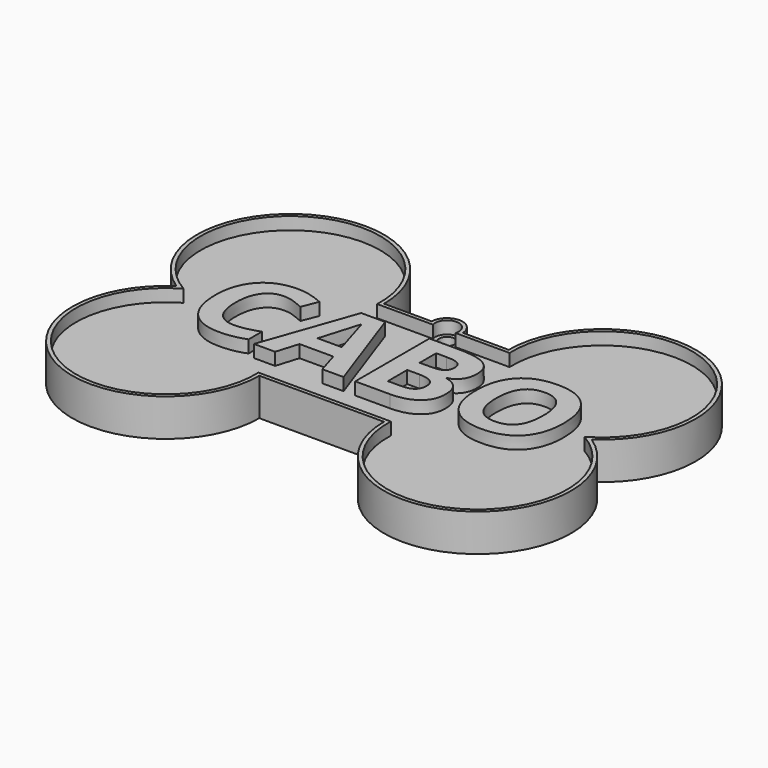
from build123d import *

# Parameters (mm, degrees)
F0_R         = 1.25
F1_DEPTH     = 4
F3_DEPTH     = 2
F4_TEXT_SIZE = 20.8333333333
F6_DEPTH     = 2


# Not quite as in the source:
# - Text() gives the source's letters only with a copy of the font that has no kerning and outlines rounded to 1/6400 em; it was checked with that copy


with BuildPart() as f1:
    # F0 (on Top) → F1 (new body)
    with BuildSketch(Plane.XY):
        with BuildLine():
            Line((-2.3552075585, 12.5), (-10, 12.5))
            ThreePointArc((-10, 12.5), (-32.0931858273, 25.7169101843), (-33.2915619759, 0))
            ThreePointArc((-33.2915619759, 0), (-32.0931858273, -25.7169101843), (-10, -12.5))
            Line((-10, -12.5), (10, -12.5))
            ThreePointArc((10, -12.5), (32.0931858273, -25.7169101843), (33.2915619759, 0))
            ThreePointArc((33.2915619759, 0), (32.0931858273, 25.7169101843), (10, 12.5))
            Line((10, 12.5), (2.6430139991, 12.5))
            ThreePointArc((2.6430139991, 12.5), (0.1439032203, 14.9333268031), (-2.3552075585, 12.5))
        make_face()
        with Locations((0.1439032203, 12.4333268031)):
            Circle(F0_R, mode=Mode.SUBTRACT)
    extrude(amount=F1_DEPTH)

    # F2 (on face) → F3 (join)
    with BuildSketch(Plane.XY.offset(4)):
        with BuildLine():
            ThreePointArc((33.2915619759, 0), (32.0931858273, 25.7169101843), (10, 12.5))
            Line((10, 12.5), (2.6430139991, 12.5))
            ThreePointArc((2.6430139991, 12.5), (0.1439032203, 14.9333268031), (-2.3552075585, 12.5))
            Line((-2.3552075585, 12.5), (-10, 12.5))
            ThreePointArc((-10, 12.5), (-32.0931858273, 25.7169101843), (-33.2915619759, 0))
            ThreePointArc((-33.2915619759, 0), (-32.0931858273, -25.7169101843), (-10, -12.5))
            Line((-10, -12.5), (10, -12.5))
            ThreePointArc((10, -12.5), (32.0931858273, -25.7169101843), (33.2915619759, 0))
        make_face()
        with BuildLine():
            ThreePointArc((-10.6125054301, -11.9), (-31.9642656137, -25.1039281362), (-32.1491258207, 0))
            ThreePointArc((-32.1491258207, 0), (-31.9642656137, 25.1039281362), (-10.6125054301, 11.9))
            Line((-10.6125054301, 11.9), (-1.6797092717, 11.9))
            ThreePointArc((-1.6797092717, 11.9), (0.1439032203, 14.3333268031), (1.9675157123, 11.9))
            Line((1.9675157123, 11.9), (10.6125054301, 11.9))
            ThreePointArc((10.6125054301, 11.9), (31.9642656137, 25.1039281362), (32.1491258207, 0))
            ThreePointArc((32.1491258207, 0), (31.9642656137, -25.1039281362), (10.6125054301, -11.9))
            Line((10.6125054301, -11.9), (-10.6125054301, -11.9))
        make_face(mode=Mode.SUBTRACT)
    extrude(amount=F3_DEPTH)

    # F4 (on face) → F6 (join)
    with BuildSketch(Plane.XY.offset(4)):
        with Locations((-29.1845703125, -6.1904743267)):
            Text('CABO', F4_TEXT_SIZE, font='Open Sans', font_style=FontStyle.BOLD, text_align=(TextAlign.LEFT, TextAlign.BOTTOM))
    extrude(amount=F6_DEPTH)


solid = f1.part
